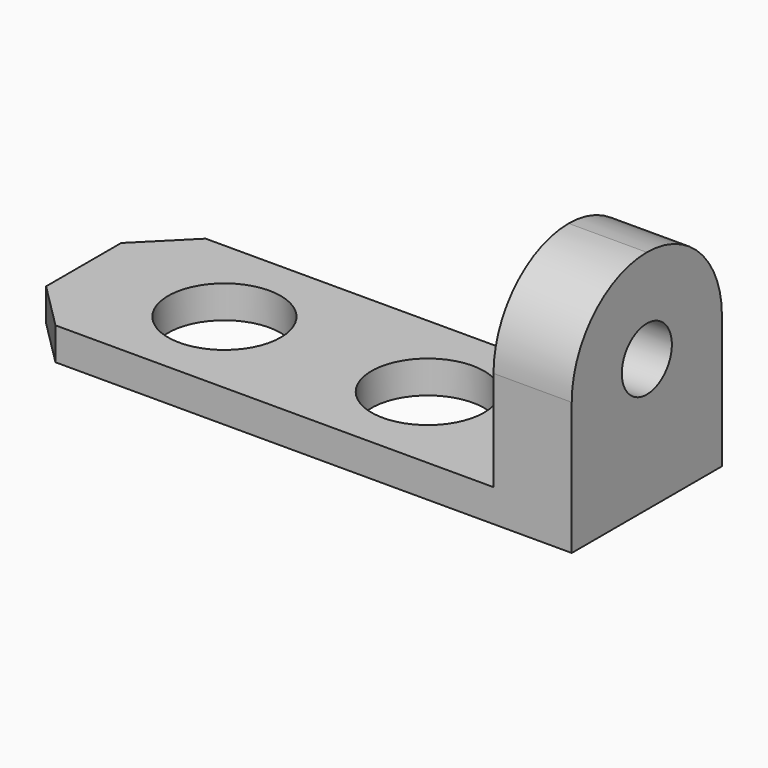
from build123d import *

# Parameters (mm, degrees)
F0_W     = 4572
F0_H     = 1524
F1_DEPTH = 264.16
F2_W     = 635
F2_H     = 1524
F3_DEPTH = 1574.8
F4_R     = 761.99999
F5_R     = 457.2
F6_DEPTH = 1475.74
F7_R     = 254
F8_DEPTH = 863.6
F9_SIZE  = 381
F10_SIZE = 381


# Not quite as in the source:
# - a fillet or chamfer is up to 0.001 mm smaller than in the source, because OpenCascade refuses the exact size


with BuildPart() as f1:
    # F0 (on Top) → F1 (new body)
    with BuildSketch(Plane.XY):
        with Locations((1.9372347742, -24.6312463946)):
            Rectangle(F0_W, F0_H)
    extrude(amount=F1_DEPTH)

    # F2 (on face) → F3 (join)
    with BuildSketch(Plane.XY.offset(264.16)):
        with Locations((1970.4372347742, -24.6312463946)):
            Rectangle(F2_W, F2_H)
    extrude(amount=F3_DEPTH)

    # F4 (radius 762 in the source; OpenCascade refuses exactly that, so slightly less here)
    f4_edges = [f1.edges().sort_by_distance(p)[0] for p in [
        (1970.437235, 737.368754, 1838.96),
        (1970.437235, -786.631246, 1838.96),
    ]]
    fillet(f4_edges, radius=F4_R)

    # F5 (on face) → F6 (cut)
    with BuildSketch(Plane.XY.offset(264.16)):
        with Locations((509.9372347742, -24.6312463946)):
            Circle(F5_R)
        with Locations((-1141.0627652258, -24.6312463946)):
            Circle(F5_R)
    extrude(amount=-F6_DEPTH, mode=Mode.SUBTRACT)

    # F7 (on face) → F8 (cut)
    with BuildSketch(Plane(origin=(1652.9372347742, 0, 0), x_dir=(0, -1, 0), z_dir=(-1, 0, 0))):
        with Locations((24.6312463946, 1076.96)):
            Circle(F7_R)
    extrude(amount=-F8_DEPTH, mode=Mode.SUBTRACT)

    # F9
    f9_edges = [f1.edges().sort_by_distance(p)[0] for p in [
        (-2284.062765, 737.368754, 132.08),
    ]]
    chamfer(f9_edges, length=F9_SIZE)

    # F10
    f10_edges = [f1.edges().sort_by_distance(p)[0] for p in [
        (-2284.062765, -786.631246, 132.08),
    ]]
    chamfer(f10_edges, length=F10_SIZE)


solid = f1.part
